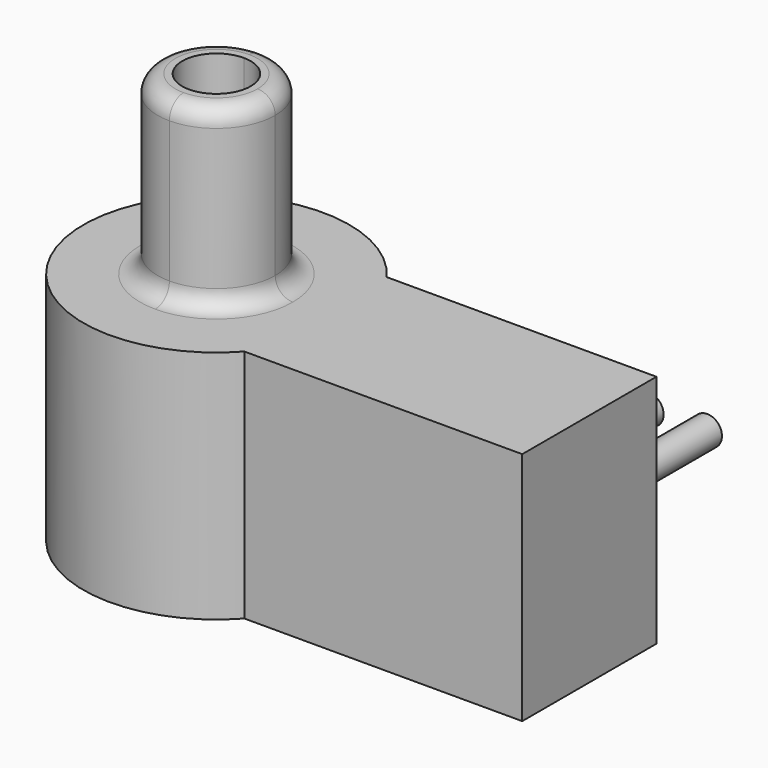
from build123d import *

# Parameters (mm, degrees)
F1_DEPTH = 70
F2_DEPTH = 40
F3_R     = 3
F4_R     = 2.5
F5_DEPTH = 25


with BuildPart() as f1:
    # F0 (on Top) → F1 (new body)
    with BuildSketch(Plane.XY):
        with BuildLine():
            ThreePointArc((-16.9023339674, 0), (-19.8312661555, 7.0710678119), (-26.9023339674, 10))
            Line((-26.9023339674, 10), (-26.9023339674, 5.8191100826))
            ThreePointArc((-26.9023339674, 5.8191100826), (-22.7876017675, 4.1147321999), (-21.0832238848, 0))
            ThreePointArc((-21.0832238848, 0), (-22.7876017675, -4.1147321999), (-26.9023339674, -5.8191100826))
            Line((-26.9023339674, -5.8191100826), (-26.9023339674, -10))
            ThreePointArc((-26.9023339674, -10), (-19.8312661555, -7.0710678119), (-16.9023339674, 0))
        make_face()
        with BuildLine():
            Line((-26.9023339674, 5.8191100826), (-26.9023339674, 10))
            ThreePointArc((-26.9023339674, 10), (-36.9023339674, 0), (-26.9023339674, -10))
            Line((-26.9023339674, -10), (-26.9023339674, -5.8191100826))
            ThreePointArc((-26.9023339674, -5.8191100826), (-32.7214440499, 0), (-26.9023339674, 5.8191100826))
        make_face()
    extrude(amount=F1_DEPTH)

    # F0 (on Top) → F2 (join)
    with BuildSketch(Plane.XY):
        with BuildLine():
            Line((37.2332856059, 13.4202644998), (21.7927563936, 13.4202644998))
            Line((21.7927563936, 13.4202644998), (-8.6679077107, 13.4202644998))
            ThreePointArc((-8.6679077107, 13.4202644998), (-5.391446413, 7.0625432229), (-4.261711181, 0))
            ThreePointArc((-4.261711181, 0), (-5.7584541043, -8.0953162068), (-10.0507873126, -15.1202901922))
            Line((-10.0507873126, -15.1202901922), (37.2332856059, -15.1202901922))
            Line((37.2332856059, -15.1202901922), (37.2332856059, 13.4202644998))
        make_face()
        with BuildLine():
            ThreePointArc((-4.261711181, 0), (-5.391446413, 7.0625432229), (-8.6679077107, 13.4202644998))
            Line((-8.6679077107, 13.4202644998), (-26.9023339674, 13.4202644998))
            Line((-26.9023339674, 13.4202644998), (-26.9023339674, 10))
            ThreePointArc((-26.9023339674, 10), (-19.8312661555, 7.0710678119), (-16.9023339674, 0))
            ThreePointArc((-16.9023339674, 0), (-19.8312661555, -7.0710678119), (-26.9023339674, -10))
            Line((-26.9023339674, -10), (-26.9023339674, -15.1202901922))
            Line((-26.9023339674, -15.1202901922), (-10.0507873126, -15.1202901922))
            ThreePointArc((-10.0507873126, -15.1202901922), (-5.7584541043, -8.0953162068), (-4.261711181, 0))
        make_face()
        with BuildLine():
            Line((-26.9023339674, 13.4202644998), (-8.6679077107, 13.4202644998))
            ThreePointArc((-8.6679077107, 13.4202644998), (-12.4988940391, 17.468220241), (-17.2027000327, 20.4576367571))
            ThreePointArc((-17.2027000327, 20.4576367571), (-49.0989219749, -4.4619817321), (-10.0507873126, -15.1202901922))
            Line((-10.0507873126, -15.1202901922), (-26.9023339674, -15.1202901922))
            Line((-26.9023339674, -15.1202901922), (-26.9023339674, -10))
            ThreePointArc((-26.9023339674, -10), (-36.9023339674, 0), (-26.9023339674, 10))
            Line((-26.9023339674, 10), (-26.9023339674, 13.4202644998))
        make_face()
    extrude(amount=F2_DEPTH)

    # F3
    f3_edges = [f1.edges().sort_by_distance(p)[0] for p in [
        (-36.902334, 0, 40),
        (-16.902334, 0, 55),
        (-36.902334, 0, 70),
    ]]
    fillet(f3_edges, radius=F3_R)

    # F4 (on face) → F5 (join)
    with BuildSketch(Plane(origin=(0, 13.4202644998, 0), x_dir=(-1, 0, 0), z_dir=(0, 1, 0))):
        with Locations((-25.8841626346, 18.0686339736)):
            Circle(F4_R)
        with Locations((-15.9560106695, 18.0668439716)):
            Circle(F4_R)
        with Locations((-7.9592689872, 16.3908023387)):
            Circle(F4_R)
        with Locations((0, 14.6713265902)):
            Circle(F4_R)
    extrude(amount=F5_DEPTH)


solid = f1.part
